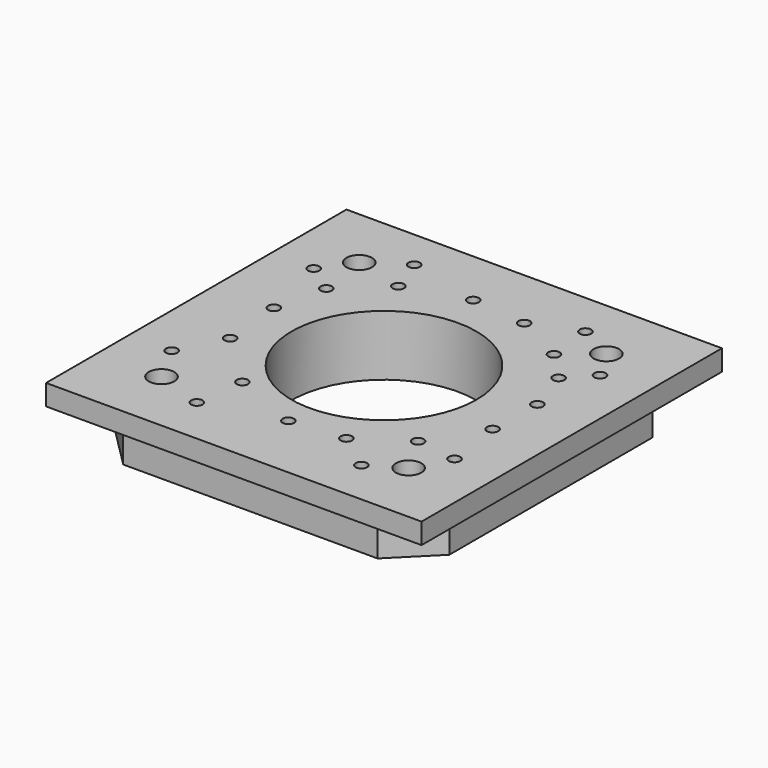
from build123d import *

# Parameters (mm, degrees)
F0_W                      = 41.9
F0_H                      = 41.9
F0_R                      = 1.6
F0_R_2                    = 11.6
F1_DEPTH                  = 5
F2_SIZE                   = 5
F3_W                      = 47.1
F3_H                      = 47.1
F3_R                      = 1.6
F3_R_2                    = 11.6
F4_DEPTH                  = 2.6
F5_R                      = 1.25
F6_DEPTH                  = 25
DRAFT_F6_DRAFTED_ANGLE    = 4
DRAFT_F6_2_DRAFTED_ANGLE  = 4
DRAFT_F6_3_DRAFTED_ANGLE  = 4
DRAFT_F6_4_DRAFTED_ANGLE  = 4
DRAFT_F6_5_DRAFTED_ANGLE  = 4
DRAFT_F6_6_DRAFTED_ANGLE  = 4
DRAFT_F6_7_DRAFTED_ANGLE  = 4
DRAFT_F6_8_DRAFTED_ANGLE  = 4
DRAFT_F6_9_DRAFTED_ANGLE  = 4
DRAFT_F6_10_DRAFTED_ANGLE = 4
DRAFT_F6_11_DRAFTED_ANGLE = 4
DRAFT_F6_12_DRAFTED_ANGLE = 4
DRAFT_F6_13_DRAFTED_ANGLE = 4
DRAFT_F6_14_DRAFTED_ANGLE = 4
DRAFT_F6_15_DRAFTED_ANGLE = 4
DRAFT_F6_16_DRAFTED_ANGLE = 4
DRAFT_F6_17_DRAFTED_ANGLE = 4
DRAFT_F6_18_DRAFTED_ANGLE = 4
DRAFT_F6_19_DRAFTED_ANGLE = 4
DRAFT_F6_20_DRAFTED_ANGLE = 4
DRAFT_F6_21_DRAFTED_ANGLE = 4
DRAFT_F6_22_DRAFTED_ANGLE = 4


# Not quite as in the source:
# - an extrude with a draft is written as a straight extrude whose walls are then drafted


with BuildPart() as f1:
    # F0 (on Top) → F1 (new body)
    with BuildSketch(Plane.XY):
        with Locations((-20.8738260887, 8.1892613277)):
            Rectangle(F0_W, F0_H)
        with Locations((-36.4238260887, -7.2607386723)):
            Circle(F0_R, mode=Mode.SUBTRACT)
        with Locations((-5.4238260887, -7.2607386723)):
            Circle(F0_R, mode=Mode.SUBTRACT)
        with Locations((-20.8738260887, 8.1892613277)):
            Circle(F0_R_2, mode=Mode.SUBTRACT)
        with Locations((-36.4238260887, 23.7392613277)):
            Circle(F0_R, mode=Mode.SUBTRACT)
        with Locations((-5.4238260887, 23.7392613277)):
            Circle(F0_R, mode=Mode.SUBTRACT)
    extrude(amount=F1_DEPTH)

    # F2
    f2_edges = [f1.edges().sort_by_distance(p)[0] for p in [
        (-41.823826, -12.760739, 2.5),
        (0.076174, -12.760739, 2.5),
        (-41.823826, 29.139261, 2.5),
        (0.076174, 29.139261, 2.5),
    ]]
    chamfer(f2_edges, length=F2_SIZE)

    # F3 (on face) → F4 (join)
    with BuildSketch(Plane.XY.offset(5)):
        with Locations((-20.8738260887, 8.1892613277)):
            Rectangle(F3_W, F3_H)
        Polygon((-36.8238260887, 29.1392613277), (-4.9238260887, 29.1392613277), (0.0761739113, 24.1392613277), (0.0761739113, -7.7607386723), (-4.9238260887, -12.7607386723), (-36.8238260887, -12.7607386723), (-41.8238260887, -7.7607386723), (-41.8238260887, 24.1392613277), align=None, mode=Mode.SUBTRACT)
        Polygon((0.0761739113, 24.1392613277), (-4.9238260887, 29.1392613277), (-36.8238260887, 29.1392613277), (-41.8238260887, 24.1392613277), (-41.8238260887, -7.7607386723), (-36.8238260887, -12.7607386723), (-4.9238260887, -12.7607386723), (0.0761739113, -7.7607386723), align=None)
        with Locations((-36.4238260887, -7.2607386723)):
            Circle(F3_R, mode=Mode.SUBTRACT)
        with Locations((-5.4238260887, -7.2607386723)):
            Circle(F3_R, mode=Mode.SUBTRACT)
        with Locations((-36.4238260887, 23.7392613277)):
            Circle(F3_R, mode=Mode.SUBTRACT)
        with Locations((-20.8738260887, 8.1892613277)):
            Circle(F3_R_2, mode=Mode.SUBTRACT)
        with Locations((-5.4238260887, 23.7392613277)):
            Circle(F3_R, mode=Mode.SUBTRACT)
    extrude(amount=F4_DEPTH)


with BuildPart() as f6_drafted:
    # F5 (on face) → F6 (new body)
    with BuildSketch(Plane(origin=(0, 0, 0), x_dir=(1, 0, 0), z_dir=(0, 0, -1))):
        with Locations((-20.8738260887, 6.8107386723)):
            Circle(F5_R)
    extrude(amount=-F6_DEPTH)

    # draft_F6_drafted
    draft_f6_drafted_walls = [f6_drafted.faces().sort_by_distance(p)[0] for p in [
        (-22.1238260887, -6.8107386723, 16.6666666667),
    ]]
    draft(draft_f6_drafted_walls, neutral_plane=Plane.XY, angle=DRAFT_F6_DRAFTED_ANGLE)


with BuildPart() as f1_1:
    add(f1.part)

    # join_F6_drafted: cut F6_drafted
    add(f6_drafted.part, mode=Mode.SUBTRACT)


with BuildPart() as f6_2_drafted:
    # F5 (on face) → F6, piece 2 (new body)
    with BuildSketch(Plane(origin=(0, 0, 0), x_dir=(1, 0, 0), z_dir=(0, 0, -1))):
        with Locations((-29.5219272375, 3.2011957373)):
            Circle(F5_R)
    extrude(amount=-F6_DEPTH)

    # draft_F6_2_drafted
    draft_f6_2_drafted_walls = [f6_2_drafted.faces().sort_by_distance(p)[0] for p in [
        (-30.7719272375, -3.2011957373, 16.6666666667),
    ]]
    draft(draft_f6_2_drafted_walls, neutral_plane=Plane.XY, angle=DRAFT_F6_2_DRAFTED_ANGLE)


with BuildPart() as f1_2:
    add(f1_1.part)

    # join_F6_2_drafted: cut F6_2_drafted
    add(f6_2_drafted.part, mode=Mode.SUBTRACT)


with BuildPart() as f6_3_drafted:
    # F5 (on face) → F6, piece 3 (new body)
    with BuildSketch(Plane(origin=(0, 0, 0), x_dir=(1, 0, 0), z_dir=(0, 0, -1))):
        with Locations((-36.2694747746, -3.3070978243)):
            Circle(F5_R)
    extrude(amount=-F6_DEPTH)

    # draft_F6_3_drafted
    draft_f6_3_drafted_walls = [f6_3_drafted.faces().sort_by_distance(p)[0] for p in [
        (-37.5194747746, 3.3070978243, 16.6666666667),
    ]]
    draft(draft_f6_3_drafted_walls, neutral_plane=Plane.XY, angle=DRAFT_F6_3_DRAFTED_ANGLE)


with BuildPart() as f1_3:
    add(f1_2.part)

    # join_F6_3_drafted: cut F6_3_drafted
    add(f6_3_drafted.part, mode=Mode.SUBTRACT)


with BuildPart() as f6_4_drafted:
    # F5 (on face) → F6, piece 4 (new body)
    with BuildSketch(Plane(origin=(0, 0, 0), x_dir=(1, 0, 0), z_dir=(0, 0, -1))):
        with Locations((-36.9536168873, -11.0101075843)):
            Circle(F5_R)
    extrude(amount=-F6_DEPTH)

    # draft_F6_4_drafted
    draft_f6_4_drafted_walls = [f6_4_drafted.faces().sort_by_distance(p)[0] for p in [
        (-38.2036168873, 11.0101075843, 16.6666666667),
    ]]
    draft(draft_f6_4_drafted_walls, neutral_plane=Plane.XY, angle=DRAFT_F6_4_DRAFTED_ANGLE)


with BuildPart() as f1_4:
    add(f1_3.part)

    # join_F6_4_drafted: cut F6_4_drafted
    add(f6_4_drafted.part, mode=Mode.SUBTRACT)


with BuildPart() as f6_5_drafted:
    # F5 (on face) → F6, piece 5 (new body)
    with BuildSketch(Plane(origin=(0, 0, 0), x_dir=(1, 0, 0), z_dir=(0, 0, -1))):
        with Locations((-35.501241684, -17.4250304699)):
            Circle(F5_R)
    extrude(amount=-F6_DEPTH)

    # draft_F6_5_drafted
    draft_f6_5_drafted_walls = [f6_5_drafted.faces().sort_by_distance(p)[0] for p in [
        (-36.751241684, 17.4250304699, 16.6666666667),
    ]]
    draft(draft_f6_5_drafted_walls, neutral_plane=Plane.XY, angle=DRAFT_F6_5_DRAFTED_ANGLE)


with BuildPart() as f1_5:
    add(f1_4.part)

    # join_F6_5_drafted: cut F6_5_drafted
    add(f6_5_drafted.part, mode=Mode.SUBTRACT)


with BuildPart() as f6_6_drafted:
    # F5 (on face) → F6, piece 6 (new body)
    with BuildSketch(Plane(origin=(0, 0, 0), x_dir=(1, 0, 0), z_dir=(0, 0, -1))):
        with Locations((-30.2926767617, -22.210393101)):
            Circle(F5_R)
    extrude(amount=-F6_DEPTH)

    # draft_F6_6_drafted
    draft_f6_6_drafted_walls = [f6_6_drafted.faces().sort_by_distance(p)[0] for p in [
        (-31.5426767617, 22.210393101, 16.6666666667),
    ]]
    draft(draft_f6_6_drafted_walls, neutral_plane=Plane.XY, angle=DRAFT_F6_6_DRAFTED_ANGLE)


with BuildPart() as f1_6:
    add(f1_5.part)

    # join_F6_6_drafted: cut F6_6_drafted
    add(f6_6_drafted.part, mode=Mode.SUBTRACT)


with BuildPart() as f6_7_drafted:
    # F5 (on face) → F6, piece 7 (new body)
    with BuildSketch(Plane(origin=(0, 0, 0), x_dir=(1, 0, 0), z_dir=(0, 0, -1))):
        with Locations((-22.7306615561, -24.4908574969)):
            Circle(F5_R)
    extrude(amount=-F6_DEPTH)

    # draft_F6_7_drafted
    draft_f6_7_drafted_walls = [f6_7_drafted.faces().sort_by_distance(p)[0] for p in [
        (-23.9806615561, 24.4908574969, 16.6666666667),
    ]]
    draft(draft_f6_7_drafted_walls, neutral_plane=Plane.XY, angle=DRAFT_F6_7_DRAFTED_ANGLE)


with BuildPart() as f1_7:
    add(f1_6.part)

    # join_F6_7_drafted: cut F6_7_drafted
    add(f6_7_drafted.part, mode=Mode.SUBTRACT)


with BuildPart() as f6_8_drafted:
    # F5 (on face) → F6, piece 8 (new body)
    with BuildSketch(Plane(origin=(0, 0, 0), x_dir=(1, 0, 0), z_dir=(0, 0, -1))):
        with Locations((-15.7743506134, -23.7953737378)):
            Circle(F5_R)
    extrude(amount=-F6_DEPTH)

    # draft_F6_8_drafted
    draft_f6_8_drafted_walls = [f6_8_drafted.faces().sort_by_distance(p)[0] for p in [
        (-17.0243506134, 23.7953737378, 16.6666666667),
    ]]
    draft(draft_f6_8_drafted_walls, neutral_plane=Plane.XY, angle=DRAFT_F6_8_DRAFTED_ANGLE)


with BuildPart() as f1_8:
    add(f1_7.part)

    # join_F6_8_drafted: cut F6_8_drafted
    add(f6_8_drafted.part, mode=Mode.SUBTRACT)


with BuildPart() as f6_9_drafted:
    # F5 (on face) → F6, piece 9 (new body)
    with BuildSketch(Plane(origin=(0, 0, 0), x_dir=(1, 0, 0), z_dir=(0, 0, -1))):
        with Locations((-9.3580633402, -20.4456690699)):
            Circle(F5_R)
    extrude(amount=-F6_DEPTH)

    # draft_F6_9_drafted
    draft_f6_9_drafted_walls = [f6_9_drafted.faces().sort_by_distance(p)[0] for p in [
        (-10.6080633402, 20.4456690699, 16.6666666667),
    ]]
    draft(draft_f6_9_drafted_walls, neutral_plane=Plane.XY, angle=DRAFT_F6_9_DRAFTED_ANGLE)


with BuildPart() as f1_9:
    add(f1_8.part)

    # join_F6_9_drafted: cut F6_9_drafted
    add(f6_9_drafted.part, mode=Mode.SUBTRACT)


with BuildPart() as f6_10_drafted:
    # F5 (on face) → F6, piece 10 (new body)
    with BuildSketch(Plane(origin=(0, 0, 0), x_dir=(1, 0, 0), z_dir=(0, 0, -1))):
        with Locations((-5.8794571087, -16.8255772442)):
            Circle(F5_R)
    extrude(amount=-F6_DEPTH)

    # draft_F6_10_drafted
    draft_f6_10_drafted_walls = [f6_10_drafted.faces().sort_by_distance(p)[0] for p in [
        (-7.1294571087, 16.8255772442, 16.6666666667),
    ]]
    draft(draft_f6_10_drafted_walls, neutral_plane=Plane.XY, angle=DRAFT_F6_10_DRAFTED_ANGLE)


with BuildPart() as f1_10:
    add(f1_9.part)

    # join_F6_10_drafted: cut F6_10_drafted
    add(f6_10_drafted.part, mode=Mode.SUBTRACT)


with BuildPart() as f6_11_drafted:
    # F5 (on face) → F6, piece 11 (new body)
    with BuildSketch(Plane(origin=(0, 0, 0), x_dir=(1, 0, 0), z_dir=(0, 0, -1))):
        with Locations((-3.9986986667, -11.1438818276)):
            Circle(F5_R)
    extrude(amount=-F6_DEPTH)

    # draft_F6_11_drafted
    draft_f6_11_drafted_walls = [f6_11_drafted.faces().sort_by_distance(p)[0] for p in [
        (-5.2486986667, 11.1438818276, 16.6666666667),
    ]]
    draft(draft_f6_11_drafted_walls, neutral_plane=Plane.XY, angle=DRAFT_F6_11_DRAFTED_ANGLE)


with BuildPart() as f1_11:
    add(f1_10.part)

    # join_F6_11_drafted: cut F6_11_drafted
    add(f6_11_drafted.part, mode=Mode.SUBTRACT)


with BuildPart() as f6_12_drafted:
    # F5 (on face) → F6, piece 12 (new body)
    with BuildSketch(Plane(origin=(0, 0, 0), x_dir=(1, 0, 0), z_dir=(0, 0, -1))):
        with Locations((-4.1490071453, -4.3147387914)):
            Circle(F5_R)
    extrude(amount=-F6_DEPTH)

    # draft_F6_12_drafted
    draft_f6_12_drafted_walls = [f6_12_drafted.faces().sort_by_distance(p)[0] for p in [
        (-5.3990071453, 4.3147387914, 16.6666666667),
    ]]
    draft(draft_f6_12_drafted_walls, neutral_plane=Plane.XY, angle=DRAFT_F6_12_DRAFTED_ANGLE)


with BuildPart() as f1_12:
    add(f1_11.part)

    # join_F6_12_drafted: cut F6_12_drafted
    add(f6_12_drafted.part, mode=Mode.SUBTRACT)


with BuildPart() as f6_13_drafted:
    # F5 (on face) → F6, piece 13 (new body)
    with BuildSketch(Plane(origin=(0, 0, 0), x_dir=(1, 0, 0), z_dir=(0, 0, -1))):
        with Locations((-8.2347663119, 2.2614069749)):
            Circle(F5_R)
    extrude(amount=-F6_DEPTH)

    # draft_F6_13_drafted
    draft_f6_13_drafted_walls = [f6_13_drafted.faces().sort_by_distance(p)[0] for p in [
        (-9.4847663119, -2.2614069749, 16.6666666667),
    ]]
    draft(draft_f6_13_drafted_walls, neutral_plane=Plane.XY, angle=DRAFT_F6_13_DRAFTED_ANGLE)


with BuildPart() as f1_13:
    add(f1_12.part)

    # join_F6_13_drafted: cut F6_13_drafted
    add(f6_13_drafted.part, mode=Mode.SUBTRACT)


with BuildPart() as f6_14_drafted:
    # F5 (on face) → F6, piece 14 (new body)
    with BuildSketch(Plane(origin=(0, 0, 0), x_dir=(1, 0, 0), z_dir=(0, 0, -1))):
        with Locations((-14.1007583588, 6.1752838083)):
            Circle(F5_R)
    extrude(amount=-F6_DEPTH)

    # draft_F6_14_drafted
    draft_f6_14_drafted_walls = [f6_14_drafted.faces().sort_by_distance(p)[0] for p in [
        (-15.3507583588, -6.1752838083, 16.6666666667),
    ]]
    draft(draft_f6_14_drafted_walls, neutral_plane=Plane.XY, angle=DRAFT_F6_14_DRAFTED_ANGLE)


with BuildPart() as f1_14:
    add(f1_13.part)

    # join_F6_14_drafted: cut F6_14_drafted
    add(f6_14_drafted.part, mode=Mode.SUBTRACT)


with BuildPart() as f6_15_drafted:
    # F5 (on face) → F6, piece 15 (new body)
    with BuildSketch(Plane(origin=(0, 0, 0), x_dir=(1, 0, 0), z_dir=(0, 0, -1))):
        with Locations((-9.4037996605, 9.6904309466)):
            Circle(F5_R)
    extrude(amount=-F6_DEPTH)

    # draft_F6_15_drafted
    draft_f6_15_drafted_walls = [f6_15_drafted.faces().sort_by_distance(p)[0] for p in [
        (-10.6537996605, -9.6904309466, 16.6666666667),
    ]]
    draft(draft_f6_15_drafted_walls, neutral_plane=Plane.XY, angle=DRAFT_F6_15_DRAFTED_ANGLE)


with BuildPart() as f1_15:
    add(f1_14.part)

    # join_F6_15_drafted: cut F6_15_drafted
    add(f6_15_drafted.part, mode=Mode.SUBTRACT)


with BuildPart() as f6_16_drafted:
    # F5 (on face) → F6, piece 16 (new body)
    with BuildSketch(Plane(origin=(0, 0, 0), x_dir=(1, 0, 0), z_dir=(0, 0, -1))):
        with Locations((-30.2965845913, 9.3706613407)):
            Circle(F5_R)
    extrude(amount=-F6_DEPTH)

    # draft_F6_16_drafted
    draft_f6_16_drafted_walls = [f6_16_drafted.faces().sort_by_distance(p)[0] for p in [
        (-31.5465845913, -9.3706613407, 16.6666666667),
    ]]
    draft(draft_f6_16_drafted_walls, neutral_plane=Plane.XY, angle=DRAFT_F6_16_DRAFTED_ANGLE)


with BuildPart() as f1_16:
    add(f1_15.part)

    # join_F6_16_drafted: cut F6_16_drafted
    add(f6_16_drafted.part, mode=Mode.SUBTRACT)


with BuildPart() as f6_17_drafted:
    # F5 (on face) → F6, piece 17 (new body)
    with BuildSketch(Plane(origin=(0, 0, 0), x_dir=(1, 0, 0), z_dir=(0, 0, -1))):
        with Locations((-39.0961505473, 2.3343011271)):
            Circle(F5_R)
    extrude(amount=-F6_DEPTH)

    # draft_F6_17_drafted
    draft_f6_17_drafted_walls = [f6_17_drafted.faces().sort_by_distance(p)[0] for p in [
        (-40.3461505473, -2.3343011271, 16.6666666667),
    ]]
    draft(draft_f6_17_drafted_walls, neutral_plane=Plane.XY, angle=DRAFT_F6_17_DRAFTED_ANGLE)


with BuildPart() as f1_17:
    add(f1_16.part)

    # join_F6_17_drafted: cut F6_17_drafted
    add(f6_17_drafted.part, mode=Mode.SUBTRACT)


with BuildPart() as f6_18_drafted:
    # F5 (on face) → F6, piece 18 (new body)
    with BuildSketch(Plane(origin=(0, 0, 0), x_dir=(1, 0, 0), z_dir=(0, 0, -1))):
        with Locations((-39.1214117408, -19.9632626027)):
            Circle(F5_R)
    extrude(amount=-F6_DEPTH)

    # draft_F6_18_drafted
    draft_f6_18_drafted_walls = [f6_18_drafted.faces().sort_by_distance(p)[0] for p in [
        (-40.3714117408, 19.9632626027, 16.6666666667),
    ]]
    draft(draft_f6_18_drafted_walls, neutral_plane=Plane.XY, angle=DRAFT_F6_18_DRAFTED_ANGLE)


with BuildPart() as f1_18:
    add(f1_17.part)

    # join_F6_18_drafted: cut F6_18_drafted
    add(f6_18_drafted.part, mode=Mode.SUBTRACT)


with BuildPart() as f6_19_drafted:
    # F5 (on face) → F6, piece 19 (new body)
    with BuildSketch(Plane(origin=(0, 0, 0), x_dir=(1, 0, 0), z_dir=(0, 0, -1))):
        with Locations((-31.9245308638, -26.7416536808)):
            Circle(F5_R)
    extrude(amount=-F6_DEPTH)

    # draft_F6_19_drafted
    draft_f6_19_drafted_walls = [f6_19_drafted.faces().sort_by_distance(p)[0] for p in [
        (-33.1745308638, 26.7416536808, 16.6666666667),
    ]]
    draft(draft_f6_19_drafted_walls, neutral_plane=Plane.XY, angle=DRAFT_F6_19_DRAFTED_ANGLE)


with BuildPart() as f1_19:
    add(f1_18.part)

    # join_F6_19_drafted: cut F6_19_drafted
    add(f6_19_drafted.part, mode=Mode.SUBTRACT)


with BuildPart() as f6_20_drafted:
    # F5 (on face) → F6, piece 20 (new body)
    with BuildSketch(Plane(origin=(0, 0, 0), x_dir=(1, 0, 0), z_dir=(0, 0, -1))):
        with Locations((-9.9625354633, -26.1413380504)):
            Circle(F5_R)
    extrude(amount=-F6_DEPTH)

    # draft_F6_20_drafted
    draft_f6_20_drafted_walls = [f6_20_drafted.faces().sort_by_distance(p)[0] for p in [
        (-11.2125354633, 26.1413380504, 16.6666666667),
    ]]
    draft(draft_f6_20_drafted_walls, neutral_plane=Plane.XY, angle=DRAFT_F6_20_DRAFTED_ANGLE)


with BuildPart() as f1_20:
    add(f1_19.part)

    # join_F6_20_drafted: cut F6_20_drafted
    add(f6_20_drafted.part, mode=Mode.SUBTRACT)


with BuildPart() as f6_21_drafted:
    # F5 (on face) → F6, piece 21 (new body)
    with BuildSketch(Plane(origin=(0, 0, 0), x_dir=(1, 0, 0), z_dir=(0, 0, -1))):
        with Locations((-3.0773431063, -19.814543426)):
            Circle(F5_R)
    extrude(amount=-F6_DEPTH)

    # draft_F6_21_drafted
    draft_f6_21_drafted_walls = [f6_21_drafted.faces().sort_by_distance(p)[0] for p in [
        (-4.3273431063, 19.814543426, 16.6666666667),
    ]]
    draft(draft_f6_21_drafted_walls, neutral_plane=Plane.XY, angle=DRAFT_F6_21_DRAFTED_ANGLE)


with BuildPart() as f1_21:
    add(f1_20.part)

    # join_F6_21_drafted: cut F6_21_drafted
    add(f6_21_drafted.part, mode=Mode.SUBTRACT)


with BuildPart() as f6_22_drafted:
    # F5 (on face) → F6, piece 22 (new body)
    with BuildSketch(Plane(origin=(0, 0, 0), x_dir=(1, 0, 0), z_dir=(0, 0, -1))):
        with Locations((-3.1061121263, 2.9601142742)):
            Circle(F5_R)
    extrude(amount=-F6_DEPTH)

    # draft_F6_22_drafted
    draft_f6_22_drafted_walls = [f6_22_drafted.faces().sort_by_distance(p)[0] for p in [
        (-4.3561121263, -2.9601142742, 16.6666666667),
    ]]
    draft(draft_f6_22_drafted_walls, neutral_plane=Plane.XY, angle=DRAFT_F6_22_DRAFTED_ANGLE)


with BuildPart() as f1_22:
    add(f1_21.part)

    # join_F6_22_drafted: cut F6_22_drafted
    add(f6_22_drafted.part, mode=Mode.SUBTRACT)


solid = f1_22.part
